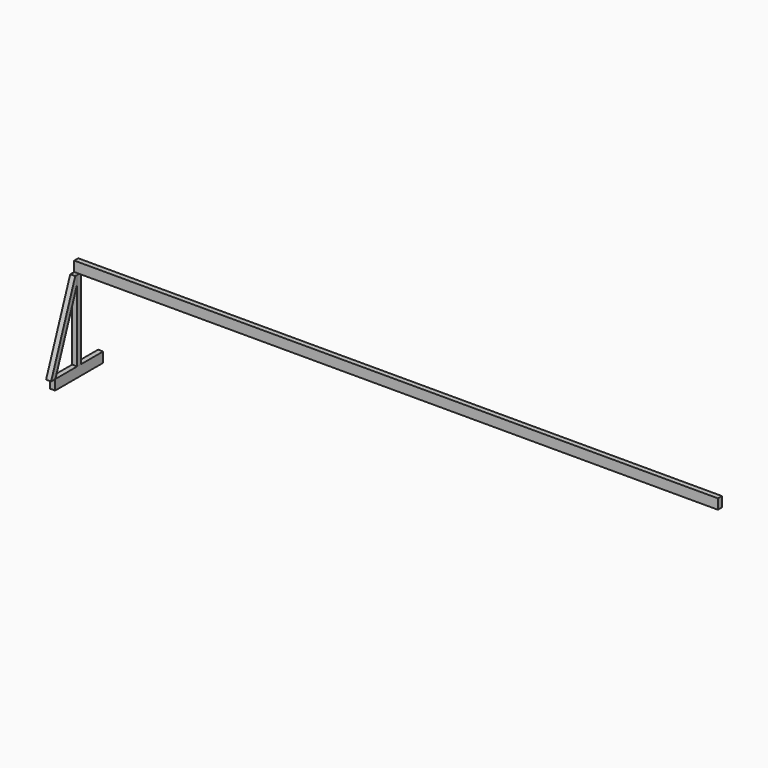
from build123d import *

# Parameters (mm, degrees)
F1_DEPTH = 406.4
F2_DEPTH = 3.175
F3_DEPTH = 3.175
F4_DEPTH = 3.175


# Not quite as in the source:
# - a feature names something its author has since deleted; it is built from what else it names


with BuildPart() as f1:
    # F0 (on Right) → F1 (new body)
    with BuildSketch(Plane.YZ):
        Polygon((20.52828, 57.15), (22.225, 57.15), (22.225, 63.4995258801), (19.05, 63.4995258801), (19.05, 57.15), align=None)
    extrude(amount=F1_DEPTH)


with BuildPart() as f2:
    # F0 (on Right) → F2 (new body)
    with BuildSketch(Plane.YZ):
        Polygon((-3.175, 6.35), (0, 6.3495258801), (0.2157236914, 6.3495258801), (17.35328, 52.0496760362), (17.35328, 57.15), (15.875, 57.15), align=None)
    extrude(amount=F2_DEPTH)


with BuildPart() as f3:
    # F0 (on Right) → F3 (new body)
    with BuildSketch(Plane.YZ):
        Polygon((0, 6.3495258801), (0, -0.0004741199), (37.88156, -0.0004741199), (37.88156, 6.3495258801), (37.4691675524, 6.3495258801), (20.52828, 6.3495258801), (18.94078, 6.3495258801), (17.35328, 6.3495258801), (0.2157236914, 6.3495258801), align=None)
    extrude(amount=F3_DEPTH)


with BuildPart() as f4:
    # F0 (on Right) → F4 (new body)
    with BuildSketch(Plane.YZ):
        Polygon((17.35328, 52.0496760362), (17.35328, 6.3495258801), (18.94078, 6.3495258801), (20.52828, 6.3495258801), (20.52828, 52.0496760362), align=None)
        Polygon((17.35328, 57.15), (17.35328, 52.0496760362), (20.52828, 52.0496760362), (20.52828, 57.15), (19.05, 57.15), align=None)
    extrude(amount=F4_DEPTH)


solid = Compound([f1.part, f2.part, f3.part, f4.part])
